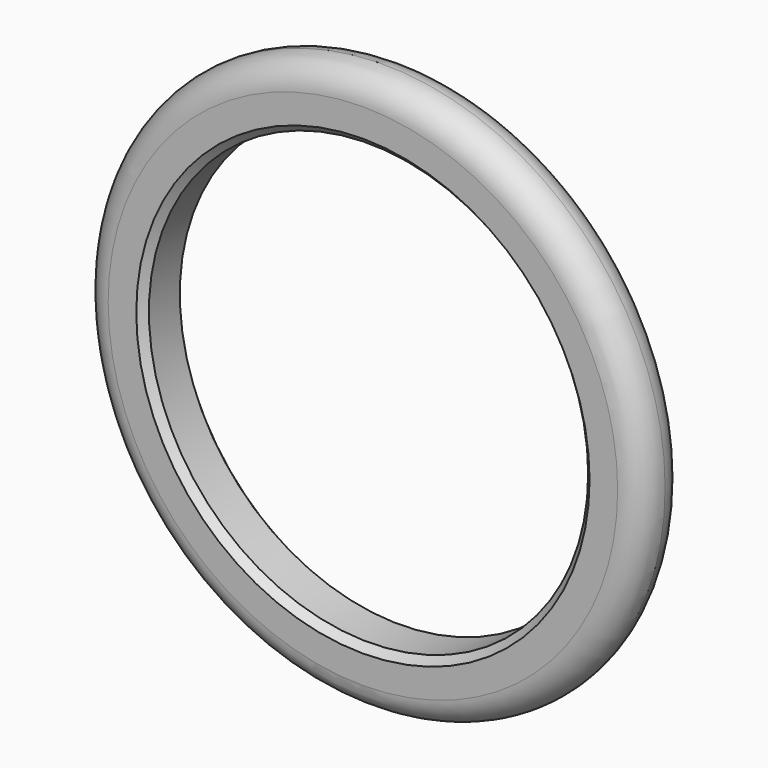
from build123d import *

# Parameters (mm, degrees)
F0_R     = 203.2
F0_R_2   = 158.75
F1_DEPTH = 38.1
F2_R     = 19.04999
F3_DEPTH = 38.1
F4_SIZE  = 5.08
F5_SIZE  = 5.08


# Not quite as in the source:
# - a fillet or chamfer is up to 0.001 mm smaller than in the source, because OpenCascade refuses the exact size


with BuildPart() as f1:
    # F0 (on Front) → F1 (new body)
    with BuildSketch(Plane.XZ):
        Circle(F0_R)
        Circle(F0_R_2, mode=Mode.SUBTRACT)
    extrude(amount=F1_DEPTH)

    # F2 (radius 19.05 in the source; OpenCascade refuses exactly that, so slightly less here)
    f2_edges = [f1.edges().sort_by_distance(p)[0] for p in [
        (-203.2, -38.1, 0),
        (-203.2, 0, 0),
    ]]
    fillet(f2_edges, radius=F2_R)

    # F3 (add): a face of the model
    f3_faces = [f1.faces().sort_by_distance(p)[0] for p in [
        (-178.9414611669, 0, 0),
    ]]
    extrude(f3_faces, amount=-F3_DEPTH)

    # F4
    f4_edges = [f1.edges().sort_by_distance(p)[0] for p in [
        (-158.75, -38.1, 0),
    ]]
    chamfer(f4_edges, length=F4_SIZE)

    # F5
    f5_edges = [f1.edges().sort_by_distance(p)[0] for p in [
        (-158.75, 0, 0),
    ]]
    chamfer(f5_edges, length=F5_SIZE)


solid = f1.part
